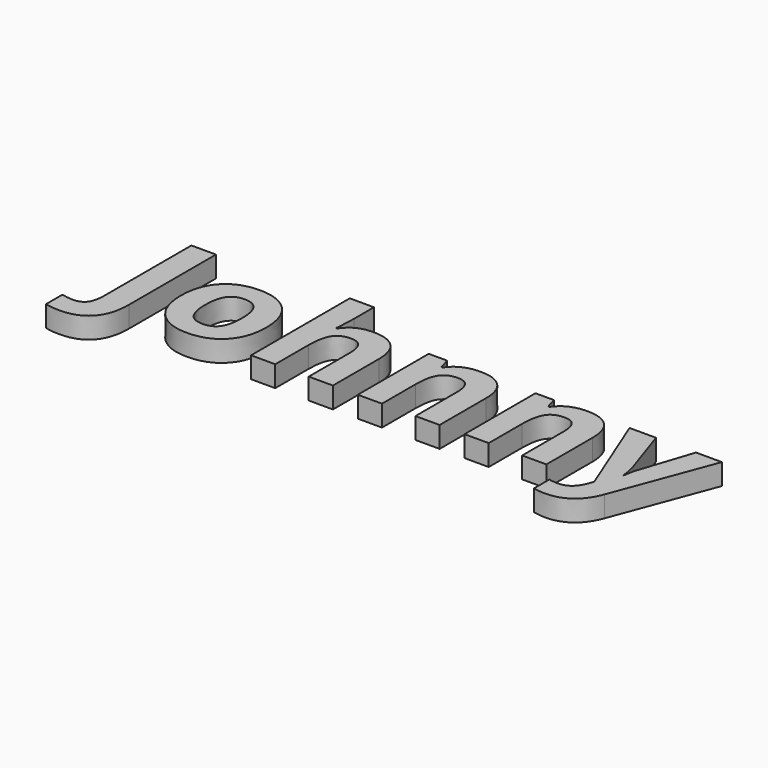
from build123d import *

# Parameters (mm, degrees)
F0_TEXT_SIZE = 58.7224546406
F1_DEPTH     = 7.62


# Not quite as in the source:
# - a feature of the source that left no trace in its solid (it failed there, or was rolled back) is left out
# - Text() gives the source's letters only with a copy of the font that has no kerning and outlines rounded to 1/6400 em; it was checked with that copy


with BuildPart() as f1:
    # F0 (on Top) → F1 (new body)
    with BuildSketch(Plane.XY):
        with Locations((-121.3885731995, -21.7386139557)):
            Text('Johnny', F0_TEXT_SIZE, font='Open Sans', font_style=FontStyle.BOLD, text_align=(TextAlign.LEFT, TextAlign.BOTTOM))
    extrude(amount=F1_DEPTH)


solid = f1.part
